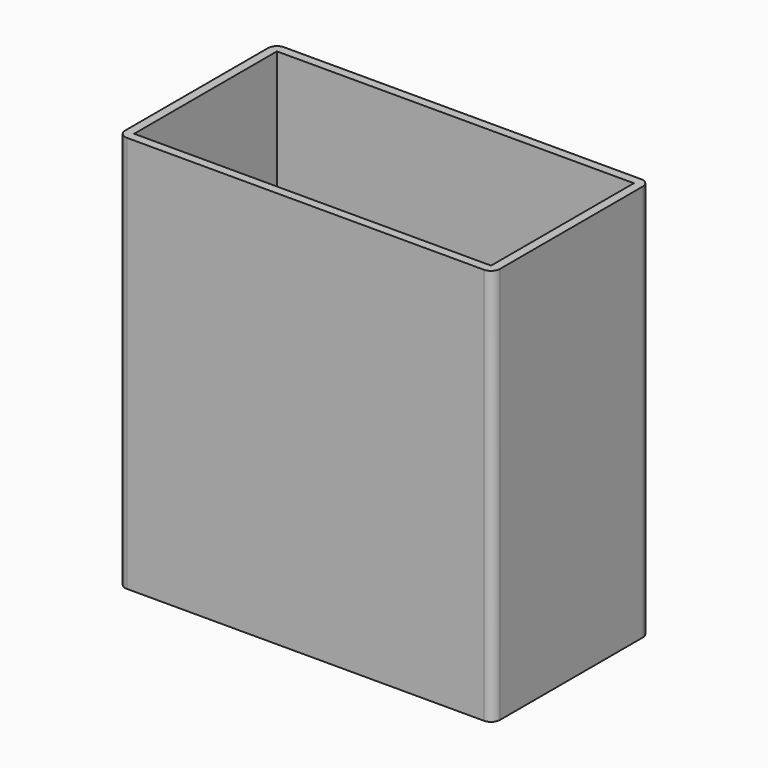
from build123d import *

# Parameters (mm, degrees)
F0_W     = 101.6
F0_H     = 50.8
F1_DEPTH = 113.03
F2_DEPTH = 6.35
F3_W     = 11.43
F3_H     = 3.175
F4_DEPTH = 63.5
F5_W     = 2.286
F5_H     = 3.175
F6_DEPTH = 63.5
F7_W     = 10.16
F7_H     = 43.18
F8_DEPTH = 73.66


# Not quite as in the source:
# - a feature names something its author has since deleted; it is built from what else it names


with BuildPart() as f1:
    # F0 (on Top) → F1 (new body)
    with BuildSketch(Plane.XY):
        with BuildLine():
            ThreePointArc((53.34, 25.4), (52.5960512242, 27.1960512242), (50.8, 27.94))
            Line((50.8, 27.94), (-50.8, 27.94))
            ThreePointArc((-50.8, 27.94), (-52.5960512242, 27.1960512242), (-53.34, 25.4))
            Line((-53.34, 25.4), (-53.34, -25.4))
            ThreePointArc((-53.34, -25.4), (-52.5960512242, -27.1960512242), (-50.8, -27.94))
            Line((-50.8, -27.94), (50.8, -27.94))
            ThreePointArc((50.8, -27.94), (52.5960512242, -27.1960512242), (53.34, -25.4))
            Line((53.34, -25.4), (53.34, 25.4))
        make_face()
        Rectangle(F0_W, F0_H, mode=Mode.SUBTRACT)
    extrude(amount=F1_DEPTH)

    # F0 (on Top) → F2 (join)
    with BuildSketch(Plane.XY):
        with BuildLine():
            ThreePointArc((53.34, 25.4), (52.5960512242, 27.1960512242), (50.8, 27.94))
            Line((50.8, 27.94), (-50.8, 27.94))
            ThreePointArc((-50.8, 27.94), (-52.5960512242, 27.1960512242), (-53.34, 25.4))
            Line((-53.34, 25.4), (-53.34, -25.4))
            ThreePointArc((-53.34, -25.4), (-52.5960512242, -27.1960512242), (-50.8, -27.94))
            Line((-50.8, -27.94), (50.8, -27.94))
            ThreePointArc((50.8, -27.94), (52.5960512242, -27.1960512242), (53.34, -25.4))
            Line((53.34, -25.4), (53.34, 25.4))
        make_face()
        Rectangle(F0_W, F0_H, mode=Mode.SUBTRACT)
        Rectangle(F0_W, F0_H)
    extrude(amount=F2_DEPTH)

    # F3 (on face) → F4 (join)
    with BuildSketch(Plane.XY.offset(6.35)):
        with Locations((-45.085, 0.1905)):
            Rectangle(F3_W, F3_H)
    extrude(amount=F4_DEPTH)

    # F5 (on face) → F6 (join)
    with BuildSketch(Plane.XY.offset(6.35)):
        with Locations((49.657, 5.3975)):
            Rectangle(F5_W, F5_H)
        with Locations((49.657, 0.1905)):
            Rectangle(F5_W, F5_H)
    extrude(amount=F6_DEPTH)

    # F7 (on Right) → F8 (cut)
    with BuildSketch(Plane.YZ):
        with Locations((5.08, 55.372)):
            Rectangle(F7_W, F7_H)
    extrude(amount=-F8_DEPTH, mode=Mode.SUBTRACT)


solid = f1.part
